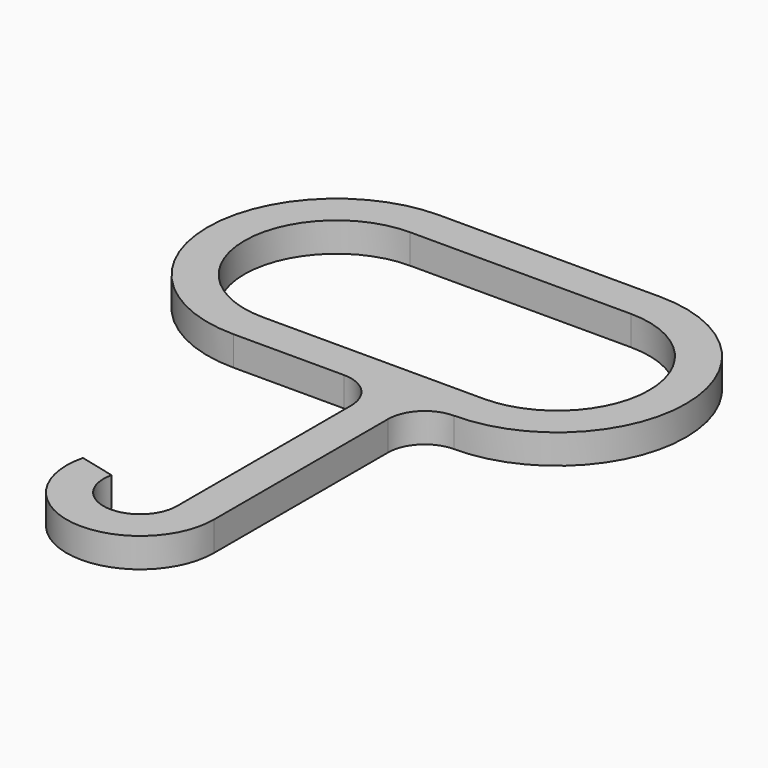
from build123d import *

# Parameters (mm, degrees)
F1_DEPTH = 4
F2_R     = 4.99999


# Not quite as in the source:
# - a fillet or chamfer is up to 0.001 mm smaller than in the source, because OpenCascade refuses the exact size


with BuildPart() as f1:
    # F0 (on Top) → F1 (new body)
    with BuildSketch(Plane.XY):
        with BuildLine():
            ThreePointArc((5, -52.0760789514), (-0.6060621786, -57.039211897), (-4.8530754543, -50.8728920851))
            Line((-4.8530754543, -50.8728920851), (-9.7061509086, -49.6697052189))
            ThreePointArc((-9.7061509086, -49.6697052189), (-1.2121243571, -62.0023448426), (10, -52.0760789514))
            Line((10, -52.0760789514), (10, -20.8603814244))
            Line((10, -20.8603814244), (10, -17.5000000745))
            Line((10, -17.5000000745), (15, -17.5000000745))
            ThreePointArc((15, -17.5000000745), (32.5000000745, 0), (15, 17.5000000745))
            Line((15, 17.5000000745), (0, 17.5000000745))
            Line((0, 17.5000000745), (-15, 17.5000000745))
            ThreePointArc((-15, 17.5000000745), (-32.5000000745, 0), (-15, -17.5000000745))
            Line((-15, -17.5000000745), (0, -17.5000000745))
            Line((0, -17.5000000745), (5, -17.5000000745))
            Line((5, -17.5000000745), (5, -18.7957836315))
            Line((5, -18.7957836315), (5, -43.4158249135))
            Line((5, -43.4158249135), (5, -52.0760789514))
        make_face()
        with BuildLine():
            ThreePointArc((-15, -12.5), (-27.5, 0), (-15, 12.5))
            Line((-15, 12.5), (0, 12.5))
            Line((0, 12.5), (15, 12.5))
            ThreePointArc((15, 12.5), (27.5, 0), (15, -12.5))
            Line((15, -12.5), (0, -12.5))
            Line((0, -12.5), (-15, -12.5))
        make_face(mode=Mode.SUBTRACT)
    extrude(amount=F1_DEPTH)

    # F2 (radius 5 in the source; OpenCascade refuses exactly that, so slightly less here)
    f2_edges = [f1.edges().sort_by_distance(p)[0] for p in [
        (5, -17.5, 2),
        (10, -17.5, 2),
    ]]
    fillet(f2_edges, radius=F2_R)


solid = f1.part
